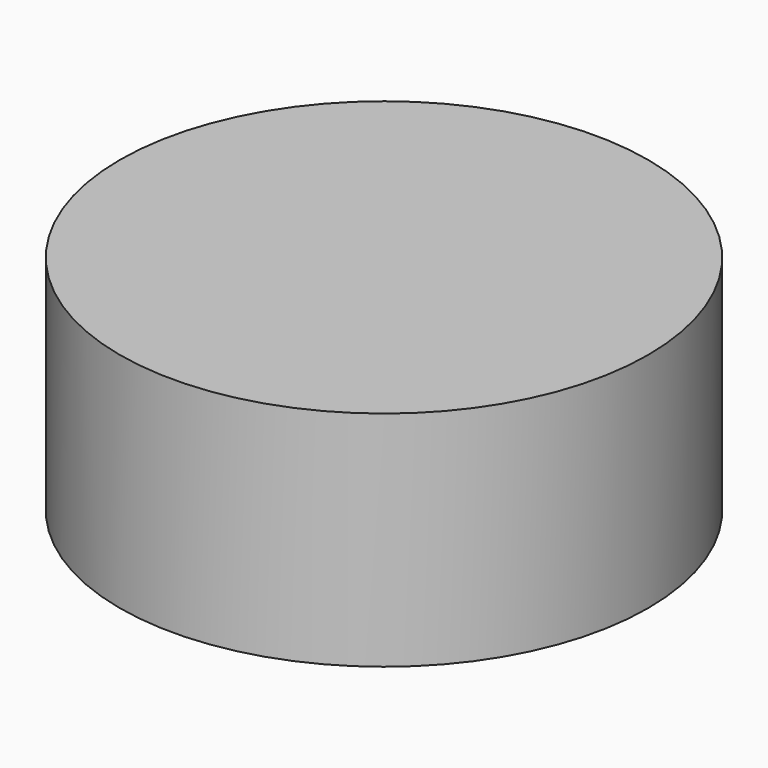
from build123d import *

# Parameters (mm, degrees)
F1_R     = 46.289516183
F3_DEPTH = 38.4330749512
F4_DEPTH = 0.635


# Not quite as in the source:
# - the program builds the solid bodies; features that only make, move or delete a surface that nothing else refers to are left out


with BuildPart() as f3:
    # F1 (on face) → F3 (new body)
    with BuildSketch(Plane.XY):
        Circle(F1_R)
    extrude(amount=-F3_DEPTH)

    # F4 (add): a face of the model
    f4_faces = [f3.faces().sort_by_distance(p)[0] for p in [
        (0, 0, -38.4330749512),
    ]]
    extrude(f4_faces, amount=F4_DEPTH)


solid = f3.part
